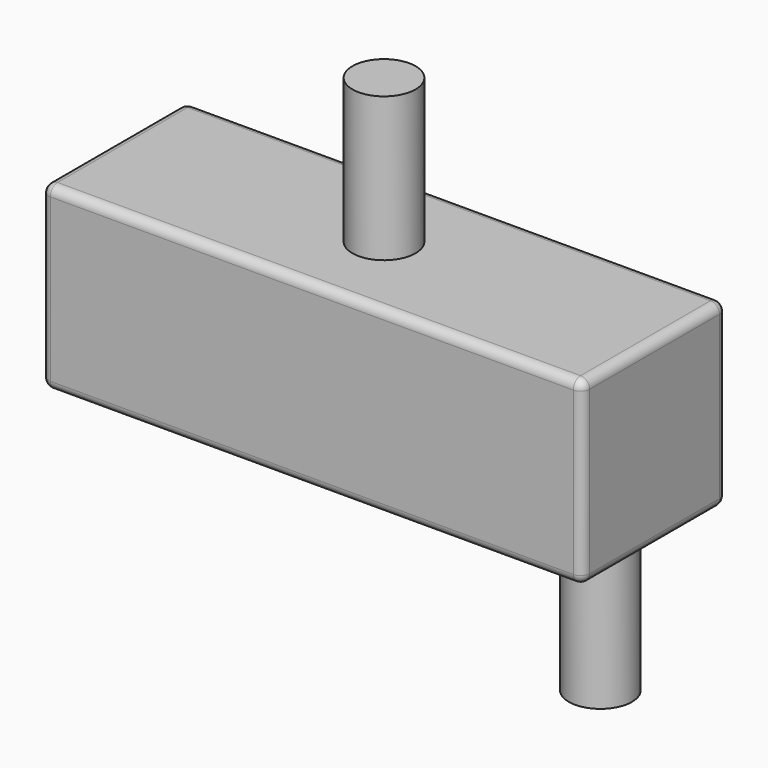
from build123d import *

# Parameters (mm, degrees)
F0_W         = 30
F0_H         = 10
F1_DEPTH     = 10
F2_R         = 1.75
F3_DEPTH     = 8
F4_R         = 1.75
F5_DEPTH     = 8
F6_R         = 0.5
F7_R         = 0.5
F8_T1_DEPTH  = 29
F8_T3_DEPTH  = 9
F8_T5_DEPTH  = 9
F8_S9_W      = 0.5
F8_S9_H      = 0.5
F8_T10_DEPTH = 0.5
F8_S15_W     = 0.5
F8_S15_H     = 0.5
F8_T16_DEPTH = 0.5
F8_S21_W     = 0.5
F8_S21_H     = 0.5
F8_T22_DEPTH = 0.5
F8_S27_W     = 0.5
F8_S27_H     = 0.5
F8_T28_DEPTH = 0.5
F8_T32_ANGLE = 90


# Not quite as in the source:
# - a fillet or chamfer that OpenCascade refuses, or shapes differently, is made with other operations: its cross-section is extruded or revolved along the edge and cut away or added


with BuildPart() as f1:
    # F0 (on Front) → F1 (new body)
    with BuildSketch(Plane.XZ):
        Rectangle(F0_W, F0_H)
    extrude(amount=-F1_DEPTH)

    # F2 (on face) → F3 (join)
    with BuildSketch(Plane.XY.offset(5)):
        with Locations((0, 5)):
            Circle(F2_R)
    extrude(amount=F3_DEPTH)

    # F4 (on face) → F5 (join)
    with BuildSketch(Plane(origin=(0, 0, -5), x_dir=(1, 0, 0), z_dir=(0, 0, -1))):
        with Locations((12, -5)):
            Circle(F4_R)
    extrude(amount=F5_DEPTH)

    # F6
    f6_edges = [f1.edges().sort_by_distance(p)[0] for p in [
        (0, 0, 5),
    ]]
    fillet(f6_edges, radius=F6_R)

    # F7
    f7_edges = [f1.edges().sort_by_distance(p)[0] for p in [
        (15, 5.25, 5),
        (-15, 5.25, 5),
        (0, 10, 5),
        (15, 5, -5),
        (15, 10, 0),
    ]]
    fillet(f7_edges, radius=F7_R)

    # F8: fillet of radius 0.5 on 3 edges, made by hand

    # F8_s2 → F8_t1 (cut)
    with BuildSketch(Plane.YZ.offset(-14.5)):
        with BuildLine():
            ThreePointArc((10, -4.5), (9.8535533906, -4.8535533906), (9.5, -5))
            Line((9.5, -5), (10, -5))
            Line((10, -5), (10, -4.5))
        make_face()
        with BuildLine():
            ThreePointArc((0, -4.5), (0.1464466094, -4.8535533906), (0.5, -5))
            Line((0.5, -5), (0, -5))
            Line((0, -5), (0, -4.5))
        make_face()
    extrude(amount=F8_T1_DEPTH, mode=Mode.SUBTRACT)

    # F8_s4 → F8_t3 (cut)
    with BuildSketch(Plane.XY.offset(-4.5)):
        with BuildLine():
            ThreePointArc((-15, 9.5), (-14.8535533906, 9.8535533906), (-14.5, 10))
            Line((-14.5, 10), (-15, 10))
            Line((-15, 10), (-15, 9.5))
        make_face()
    extrude(amount=F8_T3_DEPTH, mode=Mode.SUBTRACT)

    # F8_s6 → F8_t5 (cut)
    with BuildSketch(Plane.XZ.offset(-9.5)):
        with BuildLine():
            ThreePointArc((-15, -4.5), (-14.8535533906, -4.8535533906), (-14.5, -5))
            Line((-14.5, -5), (-15, -5))
            Line((-15, -5), (-15, -4.5))
        make_face()
    extrude(amount=F8_T5_DEPTH, mode=Mode.SUBTRACT)


with BuildPart() as f8_tool8:
    # F8_s9 → F8_t10 (new body)
    with BuildSketch(Plane.YZ.offset(-14.5)):
        with Locations((9.75, 4.75)):
            Rectangle(F8_S9_W, F8_S9_H)
    extrude(amount=-F8_T10_DEPTH)

    # F8_s11 → F8_t12 (revolve, cut)
    with BuildSketch(Plane(origin=(-14.5, 9.5, 4.5), x_dir=(0, -0.7071067812, -0.7071067812), z_dir=(0, 0.7071067812, -0.7071067812))):
        with BuildLine():
            ThreePointArc((0, -0.5), (0.5, 0), (0, 0.5))
            Line((0, 0.5), (0, -0.5))
        make_face()
    revolve(axis=Axis((-14.5, 9.5, 4.5), (-1, 0, 0)), mode=Mode.SUBTRACT)


with BuildPart() as f1_1:
    add(f1.part)

    # F8_t7: cut F8_tool8
    add(f8_tool8.part, mode=Mode.SUBTRACT)


with BuildPart() as f8_tool14:
    # F8_s15 → F8_t16 (new body)
    with BuildSketch(Plane.XZ.offset(-0.5)):
        with Locations((14.75, -4.75)):
            Rectangle(F8_S15_W, F8_S15_H)
    extrude(amount=F8_T16_DEPTH)

    # F8_s17 → F8_t18 (revolve, cut)
    with BuildSketch(Plane(origin=(14.5, 0.5, -4.5), x_dir=(-0.7071067812, 0, 0.7071067812), z_dir=(0.7071067812, 0, 0.7071067812))):
        with BuildLine():
            ThreePointArc((0, -0.5), (0.5, 0), (0, 0.5))
            Line((0, 0.5), (0, -0.5))
        make_face()
    revolve(axis=Axis((14.5, 0.5, -4.5), (0, -1, 0)), mode=Mode.SUBTRACT)


with BuildPart() as f1_2:
    add(f1_1.part)

    # F8_t13: cut F8_tool14
    add(f8_tool14.part, mode=Mode.SUBTRACT)


with BuildPart() as f8_tool20:
    # F8_s21 → F8_t22 (new body)
    with BuildSketch(Plane.XZ.offset(-9.5)):
        with Locations((14.75, -4.75)):
            Rectangle(F8_S21_W, F8_S21_H)
    extrude(amount=-F8_T22_DEPTH)

    # F8_s23 → F8_t24 (revolve, cut)
    with BuildSketch(Plane(origin=(14.5, 9.5, -4.5), x_dir=(-0.7071067812, 0, 0.7071067812), z_dir=(-0.7071067812, 0, -0.7071067812))):
        with BuildLine():
            ThreePointArc((0, -0.5), (0.5, 0), (0, 0.5))
            Line((0, 0.5), (0, -0.5))
        make_face()
    revolve(axis=Axis((14.5, 9.5, -4.5), (0, 1, 0)), mode=Mode.SUBTRACT)


with BuildPart() as f1_3:
    add(f1_2.part)

    # F8_t19: cut F8_tool20
    add(f8_tool20.part, mode=Mode.SUBTRACT)


with BuildPart() as f8_tool26:
    # F8_s27 → F8_t28 (new body)
    with BuildSketch(Plane.XY.offset(-4.5)):
        with Locations((-14.75, 9.75)):
            Rectangle(F8_S27_W, F8_S27_H)
    extrude(amount=-F8_T28_DEPTH)

    # F8_s29 → F8_t30 (revolve, cut)
    with BuildSketch(Plane(origin=(-14.5, 9.5, -4.5), x_dir=(0.7071067812, -0.7071067812, 0), z_dir=(0.7071067812, 0.7071067812, 0))):
        with BuildLine():
            ThreePointArc((0, -0.5), (0.5, 0), (0, 0.5))
            Line((0, 0.5), (0, -0.5))
        make_face()
    revolve(axis=Axis((-14.5, 9.5, -4.5), (0, 0, -1)), mode=Mode.SUBTRACT)


with BuildPart() as f1_4:
    add(f1_3.part)

    # F8_t25: cut F8_tool26
    add(f8_tool26.part, mode=Mode.SUBTRACT)

    # F8_s31 → F8_t32 (revolve, cut)
    with BuildSketch(Plane.YZ.offset(-14.5)):
        with BuildLine():
            ThreePointArc((0, -4.5), (0.1464466094, -4.8535533906), (0.5, -5))
            Line((0.5, -5), (0, -5))
            Line((0, -5), (0, -4.5))
        make_face()
    revolve(axis=Axis((-14.5, 0.5, -5), (0, 0, -1)), revolution_arc=F8_T32_ANGLE, mode=Mode.SUBTRACT)


solid = f1_4.part
